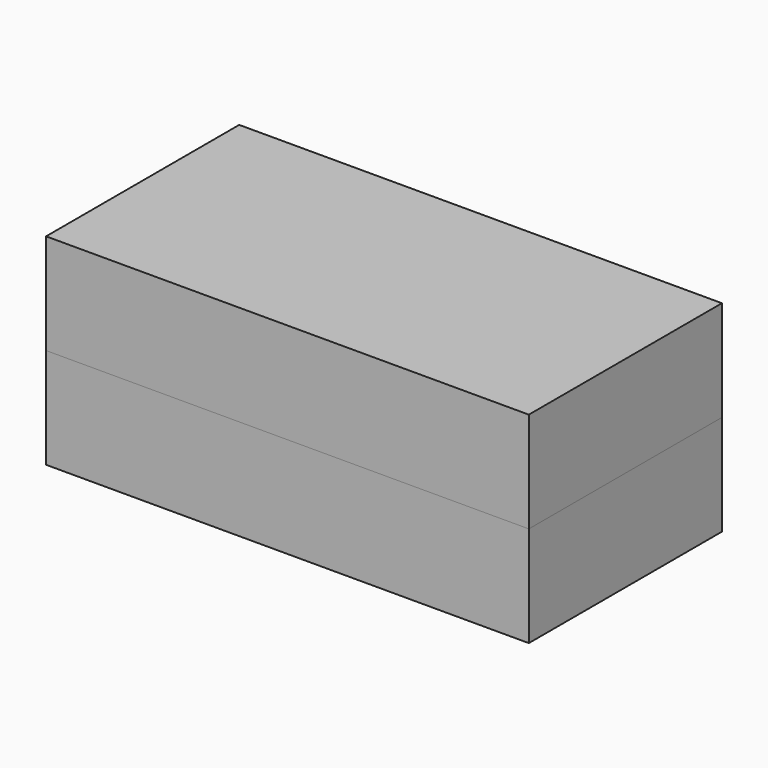
from build123d import *

# Parameters (mm, degrees)
F0_W     = 120
F0_H     = 60
F1_DEPTH = 25
F3_DEPTH = 25


# Not quite as in the source:
# - the program builds the solid bodies; features that only make, move or delete a surface that nothing else refers to are left out


with BuildPart() as f1:
    # F0 (on Top) → F1 (new body)
    with BuildSketch(Plane.XY):
        with Locations((60, 30)):
            Rectangle(F0_W, F0_H)
    extrude(amount=F1_DEPTH)


with BuildPart() as f3:
    # F3 (new): a face of the model
    f3_faces = [f1.part.faces().sort_by_distance(p)[0] for p in [
        (60, 30, 25),
    ]]
    extrude(f3_faces, amount=F3_DEPTH)


solid = Compound([f1.part, f3.part])
